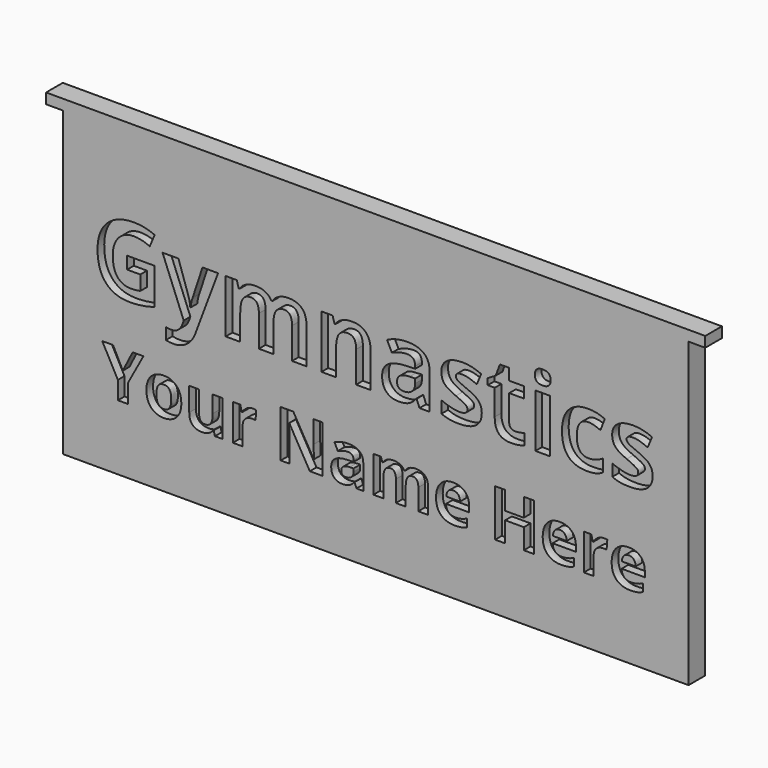
from build123d import *

# Parameters (mm, degrees)
F0_W           = 401.32
F0_H           = 190.5
F1_DEPTH       = 12.7
F2_TEXT_SIZE   = 59.4174508782
F2_TEXT_SIZE_2 = 40.1817114638
F3_DEPTH       = 5.08
F4_W           = 10.16
F4_H           = 184.15
F5_DEPTH       = 12.7


# Not quite as in the source:
# - Text() gives the source's letters only with a copy of the font that has no kerning and outlines rounded to 1/6400 em; it was checked with that copy


with BuildPart() as f1:
    # F0 (on Front) → F1 (new body)
    with BuildSketch(Plane.XZ):
        Rectangle(F0_W, F0_H)
    extrude(amount=F1_DEPTH)

    # F2 (on face) → F3 (cut)
    with BuildSketch(Plane.XZ.offset(12.7)):
        with Locations((-172.7769973204, 0)):
            Text('Gymnastics', F2_TEXT_SIZE, font='Open Sans', font_style=FontStyle.BOLD, text_align=(TextAlign.LEFT, TextAlign.BOTTOM))
        with Locations((-166.472800076, -55.549918296)):
            Text('Your Name Here', F2_TEXT_SIZE_2, font='Open Sans', font_style=FontStyle.BOLD, text_align=(TextAlign.LEFT, TextAlign.BOTTOM))
    extrude(amount=-F3_DEPTH, mode=Mode.SUBTRACT)

    # F4 (on face) → F5 (cut)
    with BuildSketch(Plane.XZ.offset(12.7)):
        with Locations((-195.58, -3.175)):
            Rectangle(F4_W, F4_H)
        with Locations((195.58, -3.175)):
            Rectangle(F4_W, F4_H)
    extrude(amount=-F5_DEPTH, mode=Mode.SUBTRACT)


solid = f1.part
